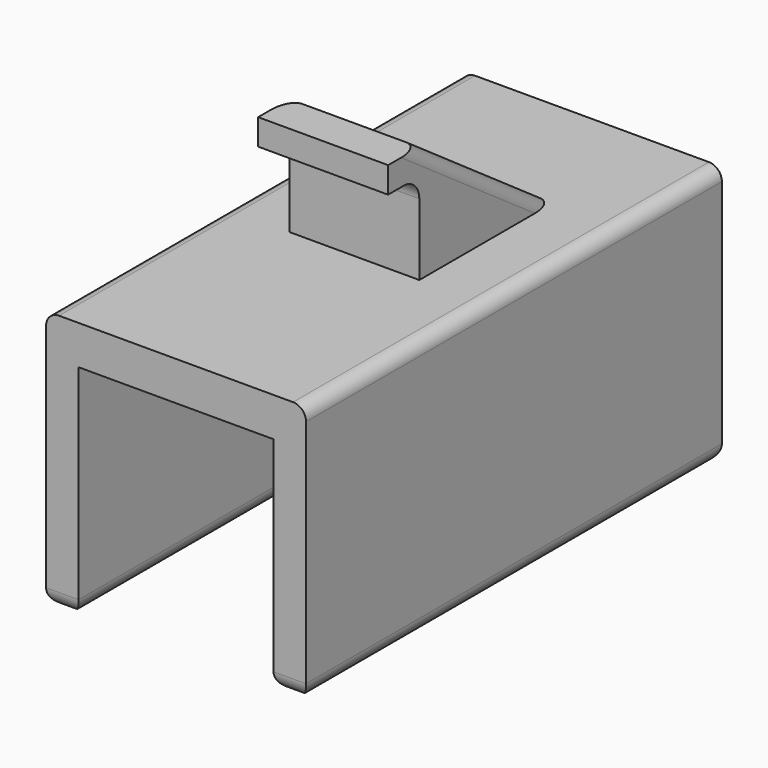
from build123d import *

# Parameters (mm, degrees)
F1_DEPTH      = 101.6
F2_R          = 3.17499
F3_R          = 3.17499
F5_DEPTH      = 12.7
F5_DEPTH_BACK = 12.7
F6_R          = 2.54
F7_R          = 2.54
F8_R          = 2.54
F9_R          = 2.54
F10_R         = 3.81


# Not quite as in the source:
# - a fillet or chamfer is up to 0.001 mm smaller than in the source, because OpenCascade refuses the exact size


with BuildPart() as f1:
    # F0 (on Front) → F1 (new body)
    with BuildSketch(Plane.XZ):
        Polygon((-25.4, 25.4), (-25.4, -25.4), (-19.05, -25.4), (-19.05, 17.78), (19.05, 17.78), (19.05, -25.4), (25.4, -25.4), (25.4, 25.4), align=None)
    extrude(amount=F1_DEPTH)

    # F2 (radius 3.175 in the source; OpenCascade refuses exactly that, so slightly less here)
    f2_edges = [f1.edges().sort_by_distance(p)[0] for p in [
        (-25.4, -50.8, -25.4),
        (-19.05, -50.8, -25.4),
        (-22.225, 0, -25.4),
        (-22.225, -101.6, -25.4),
    ]]
    fillet(f2_edges, radius=F2_R)

    # F3 (radius 3.175 in the source; OpenCascade refuses exactly that, so slightly less here)
    f3_edges = [f1.edges().sort_by_distance(p)[0] for p in [
        (19.05, -50.8, -25.4),
        (25.4, -50.8, -25.4),
        (22.225, 0, -25.4),
        (22.225, -101.6, -25.4),
    ]]
    fillet(f3_edges, radius=F3_R)

    # F4 (on Right) → F5 (join, two sides)
    with BuildSketch(Plane.YZ) as f5_sk:
        Polygon((-58.0474634341, 25.4), (-25.4, 25.4), (-58.0474634341, 48.26), (-65.6674634341, 48.26), (-65.6674634341, 43.18), (-58.0474634341, 43.18), align=None)
    extrude(amount=F5_DEPTH)
    extrude(f5_sk.sketch, amount=-F5_DEPTH_BACK)

    # F6
    f6_edges = [f1.edges().sort_by_distance(p)[0] for p in [
        (25.4, -50.8, 25.4),
    ]]
    fillet(f6_edges, radius=F6_R)

    # F7
    f7_edges = [f1.edges().sort_by_distance(p)[0] for p in [
        (-25.4, -50.8, 25.4),
    ]]
    fillet(f7_edges, radius=F7_R)

    # F8
    f8_edges = [f1.edges().sort_by_distance(p)[0] for p in [
        (-12.7, -41.723732, 36.83),
    ]]
    fillet(f8_edges, radius=F8_R)

    # F9
    f9_edges = [f1.edges().sort_by_distance(p)[0] for p in [
        (12.7, -41.723732, 36.83),
    ]]
    fillet(f9_edges, radius=F9_R)

    # F10
    f10_edges = [f1.edges().sort_by_distance(p)[0] for p in [
        (0, -58.047463, 43.18),
    ]]
    fillet(f10_edges, radius=F10_R)


solid = f1.part
